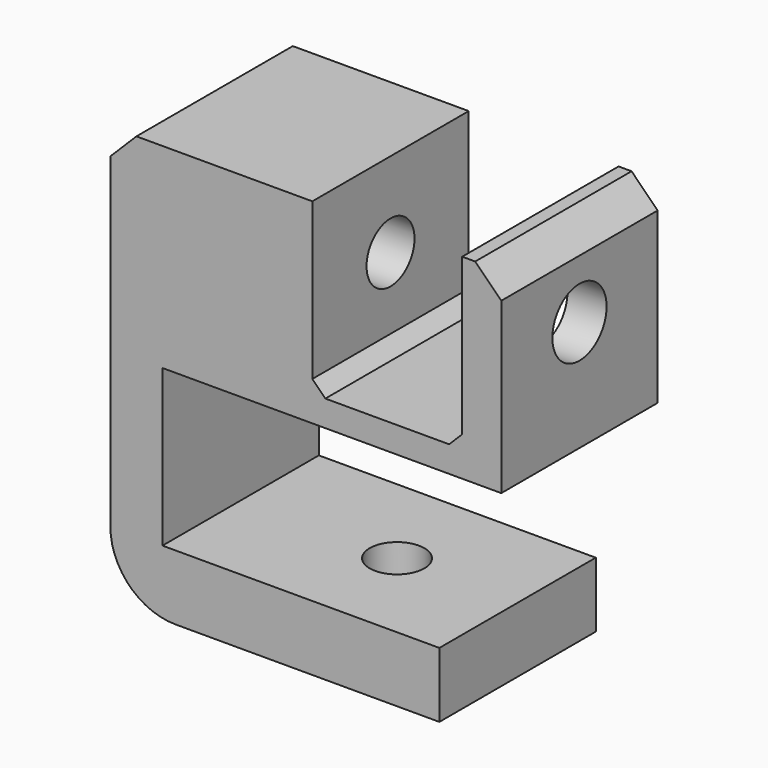
from build123d import *

# Parameters (mm, degrees)
F1_DEPTH = 15
F2_SIZE  = 2
F3_SIZE  = 1
F4_R     = 2.1
F5_DEPTH = 5
F6_R     = 2.3
F7_DEPTH = 29.5
F8_R     = 2.6
F8_R_2   = 2.3
F9_DEPTH = 3


with BuildPart() as f1:
    # F0 (on Front) → F1 (new body)
    with BuildSketch(Plane.XZ):
        with BuildLine():
            Line((0, 32), (0, 5))
            ThreePointArc((0, 5), (1.4644660941, 1.4644660941), (5, 0))
            Line((5, 0), (25.25, 0))
            Line((25.25, 0), (25.25, 5))
            Line((25.25, 5), (4, 5))
            Line((4, 5), (4, 17))
            Line((4, 17), (30, 17))
            Line((30, 17), (30, 32))
            Line((30, 32), (27, 32))
            Line((27, 32), (27, 19))
            Line((27, 19), (15.5, 19))
            Line((15.5, 19), (15.5, 32))
            Line((15.5, 32), (0, 32))
        make_face()
    extrude(amount=F1_DEPTH)

    # F2
    f2_edges = [f1.edges().sort_by_distance(p)[0] for p in [
        (0, -7.5, 32),
        (30, -7.5, 32),
    ]]
    chamfer(f2_edges, length=F2_SIZE)

    # F3
    f3_edges = [f1.edges().sort_by_distance(p)[0] for p in [
        (15.5, -7.5, 19),
        (27, -7.5, 19),
    ]]
    chamfer(f3_edges, length=F3_SIZE)

    # F4 (on face) → F5 (cut, through all)
    with BuildSketch(Plane(origin=(0, 0, 0), x_dir=(1, 0, 0), z_dir=(0, 0, -1))):
        with Locations((16, 7.5)):
            Circle(F4_R)
    extrude(amount=-F5_DEPTH, mode=Mode.SUBTRACT)

    # F6 (on face) → F7 (cut)
    with BuildSketch(Plane.YZ.offset(30)):
        with Locations((-7.5, 25.5)):
            Circle(F6_R)
    extrude(amount=-F7_DEPTH, mode=Mode.SUBTRACT)

    # F8 (on face) → F9 (cut, through all)
    with BuildSketch(Plane.YZ.offset(30)):
        with Locations((-7.5, 25.5)):
            Circle(F8_R)
        with Locations((-7.5, 25.5)):
            Circle(F8_R_2, mode=Mode.SUBTRACT)
    extrude(amount=-F9_DEPTH, mode=Mode.SUBTRACT)


solid = f1.part
